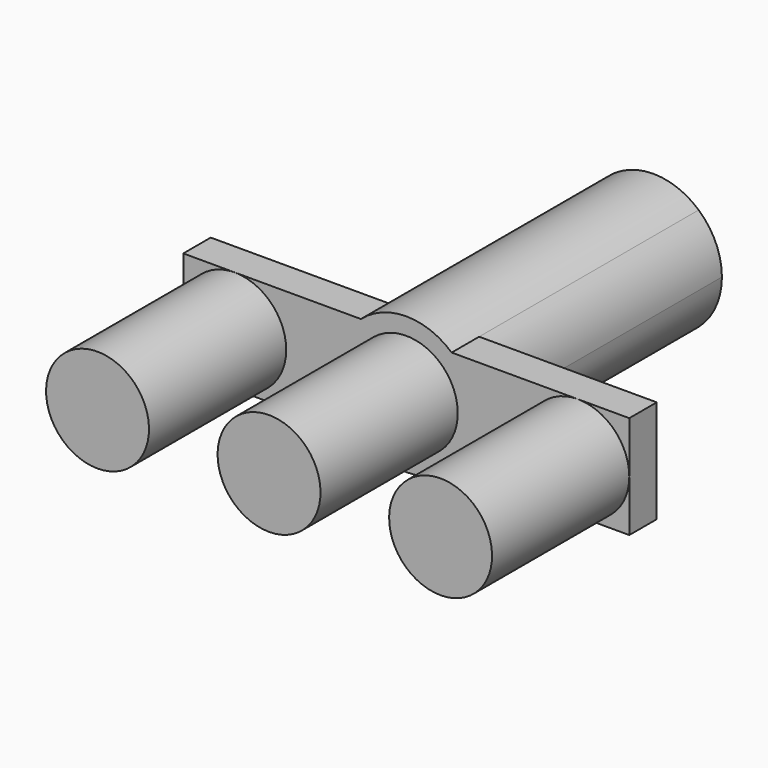
from build123d import *

# Parameters (mm, degrees)
F1_DEPTH = 5
F2_DEPTH = 30
F3_DEPTH = 40


# Not quite as in the source:
# - after a boolean that leaves OpenCascade's solid faulty, fix() repairs it


with BuildPart() as f1:
    # F0 (on Front) → F1 (new body)
    with BuildSketch(Plane.XZ):
        with BuildLine():
            Line((-25, 7.5), (-32.5, 7.5))
            Line((-32.5, 7.5), (-32.5, 0))
            ThreePointArc((-32.5, 0), (-30.3033008589, 5.3033008589), (-25, 7.5))
        make_face()
        with BuildLine():
            Line((-6.6143782777, 7.5), (-25, 7.5))
            ThreePointArc((-25, 7.5), (-19.6966991411, 5.3033008589), (-17.5, 0))
            ThreePointArc((-17.5, 0), (-19.6966991411, -5.3033008589), (-25, -7.5))
            Line((-25, -7.5), (-6.6143782777, -7.5))
            ThreePointArc((-6.6143782777, -7.5), (-10, 0), (-6.6143782777, 7.5))
        make_face()
        with BuildLine():
            ThreePointArc((-17.5, 0), (-19.6966991411, 5.3033008589), (-25, 7.5))
            ThreePointArc((-25, 7.5), (-30.3033008589, 5.3033008589), (-32.5, 0))
            ThreePointArc((-32.5, 0), (-30.3033008589, -5.3033008589), (-25, -7.5))
            ThreePointArc((-25, -7.5), (-19.6966991411, -5.3033008589), (-17.5, 0))
        make_face()
        with BuildLine():
            ThreePointArc((-25, -7.5), (-30.3033008589, -5.3033008589), (-32.5, 0))
            Line((-32.5, 0), (-32.5, -7.5))
            Line((-32.5, -7.5), (-25, -7.5))
        make_face()
        with BuildLine():
            ThreePointArc((6.6143782777, 7.5), (0, 10), (-6.6143782777, 7.5))
            Line((-6.6143782777, 7.5), (0, 7.5))
            Line((0, 7.5), (6.6143782777, 7.5))
        make_face()
        with BuildLine():
            Line((0, 7.5), (-6.6143782777, 7.5))
            ThreePointArc((-6.6143782777, 7.5), (-10, 0), (-6.6143782777, -7.5))
            Line((-6.6143782777, -7.5), (-2.86e-08, -7.5))
            ThreePointArc((-2.86e-08, -7.5), (-7.5, 1.43e-08), (0, 7.5))
        make_face()
        with BuildLine():
            Line((6.6143782777, 7.5), (0, 7.5))
            ThreePointArc((0, 7.5), (5.3033008589, 5.3033008589), (7.5, 0))
            ThreePointArc((7.5, 0), (5.3033008488, -5.303300869), (-2.86e-08, -7.5))
            Line((-2.86e-08, -7.5), (6.6143782777, -7.5))
            ThreePointArc((6.6143782777, -7.5), (9.1143782777, -4.1143782777), (10, 0))
            ThreePointArc((10, 0), (9.1143782777, 4.1143782777), (6.6143782777, 7.5))
        make_face()
        with BuildLine():
            Line((25, 7.5), (6.6143782777, 7.5))
            ThreePointArc((6.6143782777, 7.5), (9.1143782777, 4.1143782777), (10, 0))
            ThreePointArc((10, 0), (9.1143782777, -4.1143782777), (6.6143782777, -7.5))
            Line((6.6143782777, -7.5), (25, -7.5))
            ThreePointArc((25, -7.5), (17.5, 0), (25, 7.5))
        make_face()
        with BuildLine():
            Line((-2.86e-08, -7.5), (-6.6143782777, -7.5))
            ThreePointArc((-6.6143782777, -7.5), (0, -10), (6.6143782777, -7.5))
            Line((6.6143782777, -7.5), (-2.86e-08, -7.5))
        make_face()
        with BuildLine():
            Line((32.5, 7.5), (25, 7.5))
            ThreePointArc((25, 7.5), (30.3033008589, 5.3033008589), (32.5, 0))
            Line((32.5, 0), (32.5, 7.5))
        make_face()
        with BuildLine():
            ThreePointArc((32.5, 0), (30.3033008589, 5.3033008589), (25, 7.5))
            ThreePointArc((25, 7.5), (17.5, 0), (25, -7.5))
            ThreePointArc((25, -7.5), (30.3033008589, -5.3033008589), (32.5, 0))
        make_face()
        with BuildLine():
            Line((32.5, -7.5), (32.5, 0))
            ThreePointArc((32.5, 0), (30.3033008589, -5.3033008589), (25, -7.5))
            Line((25, -7.5), (32.5, -7.5))
        make_face()
    extrude(amount=F1_DEPTH)

    # F0 (on Front) → F2 (join)
    with BuildSketch(Plane.XZ):
        with BuildLine():
            ThreePointArc((7.5, 0), (5.3033008589, 5.3033008589), (0, 7.5))
            ThreePointArc((0, 7.5), (-7.5, 1.43e-08), (-2.86e-08, -7.5))
            ThreePointArc((-2.86e-08, -7.5), (5.3033008488, -5.303300869), (7.5, 0))
        make_face()
        with BuildLine():
            ThreePointArc((32.5, 0), (30.3033008589, 5.3033008589), (25, 7.5))
            ThreePointArc((25, 7.5), (17.5, 0), (25, -7.5))
            ThreePointArc((25, -7.5), (30.3033008589, -5.3033008589), (32.5, 0))
        make_face()
        with BuildLine():
            ThreePointArc((-17.5, 0), (-19.6966991411, 5.3033008589), (-25, 7.5))
            ThreePointArc((-25, 7.5), (-30.3033008589, 5.3033008589), (-32.5, 0))
            ThreePointArc((-32.5, 0), (-30.3033008589, -5.3033008589), (-25, -7.5))
            ThreePointArc((-25, -7.5), (-19.6966991411, -5.3033008589), (-17.5, 0))
        make_face()
    extrude(amount=F2_DEPTH)

    # F0 (on Front) → F3 (join)
    with BuildSketch(Plane.XZ):
        with BuildLine():
            Line((0, 7.5), (-6.6143782777, 7.5))
            ThreePointArc((-6.6143782777, 7.5), (-10, 0), (-6.6143782777, -7.5))
            Line((-6.6143782777, -7.5), (-2.86e-08, -7.5))
            ThreePointArc((-2.86e-08, -7.5), (-7.5, 1.43e-08), (0, 7.5))
        make_face()
        with BuildLine():
            ThreePointArc((7.5, 0), (5.3033008589, 5.3033008589), (0, 7.5))
            ThreePointArc((0, 7.5), (-7.5, 1.43e-08), (-2.86e-08, -7.5))
            ThreePointArc((-2.86e-08, -7.5), (5.3033008488, -5.303300869), (7.5, 0))
        make_face()
        with BuildLine():
            Line((-2.86e-08, -7.5), (-6.6143782777, -7.5))
            ThreePointArc((-6.6143782777, -7.5), (0, -10), (6.6143782777, -7.5))
            Line((6.6143782777, -7.5), (-2.86e-08, -7.5))
        make_face()
        with BuildLine():
            Line((6.6143782777, 7.5), (0, 7.5))
            ThreePointArc((0, 7.5), (5.3033008589, 5.3033008589), (7.5, 0))
            ThreePointArc((7.5, 0), (5.3033008488, -5.303300869), (-2.86e-08, -7.5))
            Line((-2.86e-08, -7.5), (6.6143782777, -7.5))
            ThreePointArc((6.6143782777, -7.5), (9.1143782777, -4.1143782777), (10, 0))
            ThreePointArc((10, 0), (9.1143782777, 4.1143782777), (6.6143782777, 7.5))
        make_face()
        with BuildLine():
            ThreePointArc((6.6143782777, 7.5), (0, 10), (-6.6143782777, 7.5))
            Line((-6.6143782777, 7.5), (0, 7.5))
            Line((0, 7.5), (6.6143782777, 7.5))
        make_face()
    extrude(amount=-F3_DEPTH)

    add(f1.part.fix(), mode=Mode.REPLACE)


solid = f1.part
